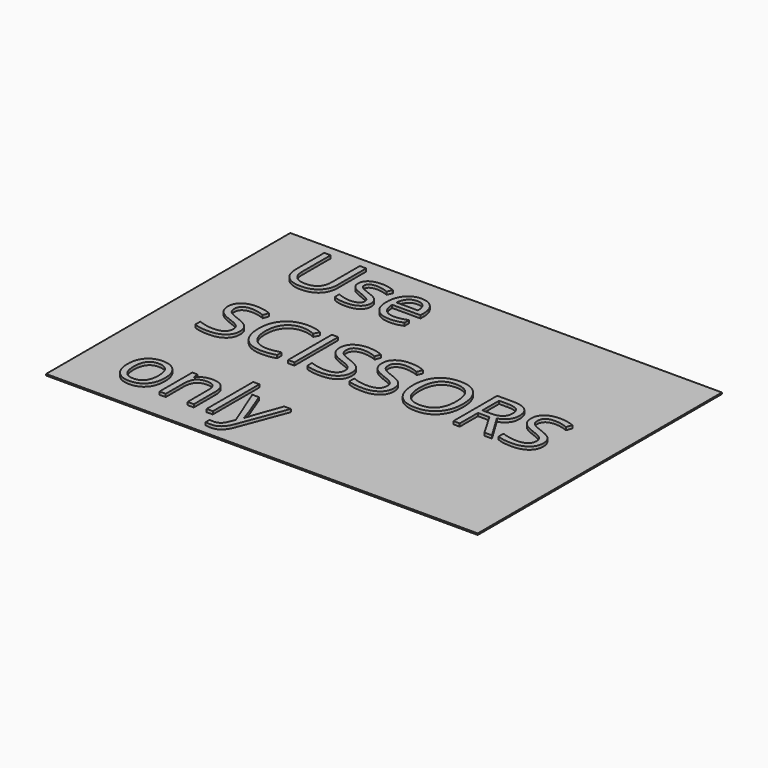
from build123d import *

# Parameters (mm, degrees)
F0_W         = 297
F0_H         = 210
F1_DEPTH     = 1
F2_TEXT_SIZE = 52.7777777778
F3_DEPTH     = 2


# Not quite as in the source:
# - Text() gives the source's letters only with a copy of the font that has no kerning and outlines rounded to 1/6400 em; it was checked with that copy


with BuildPart() as f1:
    # F0 (on Top) → F1 (new body)
    with BuildSketch(Plane.XY):
        with Locations((-110.8175859451, 85.8470010757)):
            Rectangle(F0_W, F0_H)
    extrude(amount=F1_DEPTH)

    # F2 (on face) → F3 (join)
    with BuildSketch(Plane.XY.offset(1)):
        with Locations((-232.9810586871, 143.4949366924)):
            Text('Use', F2_TEXT_SIZE, font='Open Sans', text_align=(TextAlign.LEFT, TextAlign.BOTTOM))
        with Locations((-232.9810586871, 71.7171589146)):
            Text('SCISSORS', F2_TEXT_SIZE, font='Open Sans', text_align=(TextAlign.LEFT, TextAlign.BOTTOM))
        with Locations((-232.9810586871, -0.0606188632)):
            Text('only', F2_TEXT_SIZE, font='Open Sans', text_align=(TextAlign.LEFT, TextAlign.BOTTOM))
    extrude(amount=F3_DEPTH)


solid = f1.part
